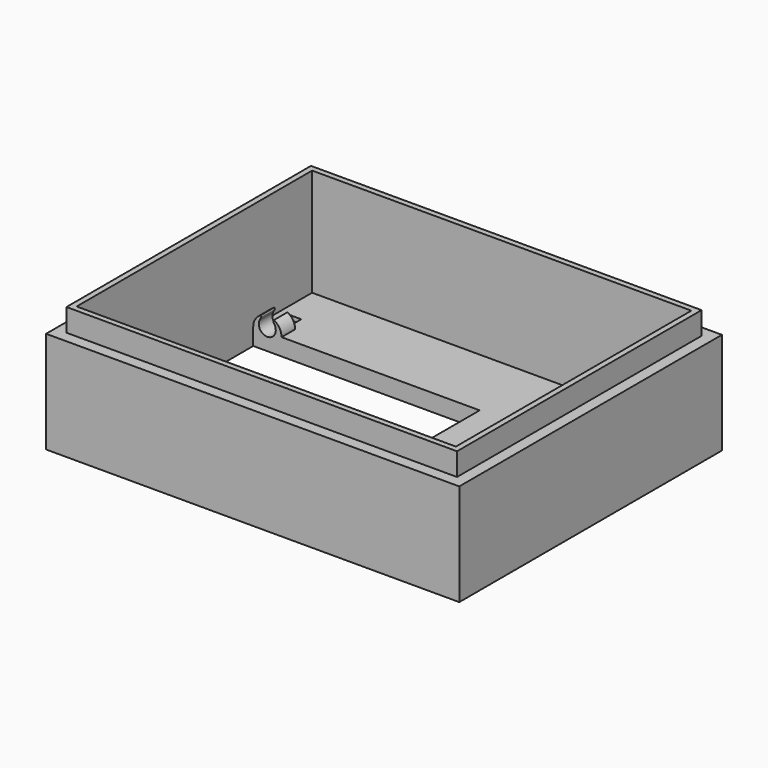
from build123d import *

# Parameters (mm, degrees)
F0_W      = 73
F0_H      = 22
F1_DEPTH  = 29
F2_W      = 67
F2_H      = 52
F3_DEPTH  = 19
F4_W      = 58
F4_H      = 4
F5_DEPTH  = 2
F6_W      = 71
F6_H      = 4
F7_DEPTH  = 2
F8_W      = 56
F8_H      = 4
F9_DEPTH  = 2
F10_W     = 69
F10_H     = 4
F11_DEPTH = 2
F12_W     = 42
F12_H     = 28
F13_DEPTH = 22.001
F14_W     = 2.5
F14_H     = 3
F16_W     = 2.5
F16_H     = 3
F18_R     = 1.5
F19_DEPTH = 35.32766
F20_DEPTH = 5.87666
F22_DEPTH = 38.628
F23_W     = 28
F23_H     = 1.5
F24_DEPTH = 2


with BuildPart() as f1:
    # F0 (on Front) → F1 (new body, symmetric)
    with BuildSketch(Plane.XZ):
        Rectangle(F0_W, F0_H)
    extrude(amount=F1_DEPTH, both=True)

    # F2 (on face) → F3 (cut)
    with BuildSketch(Plane.XY.offset(11)):
        Rectangle(F2_W, F2_H)
    extrude(amount=-F3_DEPTH, mode=Mode.SUBTRACT)

    # F4 (on face) → F5 (cut)
    with BuildSketch(Plane.YZ.offset(36.5)):
        with Locations((0, 9)):
            Rectangle(F4_W, F4_H)
    extrude(amount=-F5_DEPTH, mode=Mode.SUBTRACT)

    # F6 (on face) → F7 (cut)
    with BuildSketch(Plane.XZ.offset(29)):
        with Locations((-1, 9)):
            Rectangle(F6_W, F6_H)
    extrude(amount=-F7_DEPTH, mode=Mode.SUBTRACT)

    # F8 (on face) → F9 (cut)
    with BuildSketch(Plane(origin=(-36.5, 0, 0), x_dir=(0, -1, 0), z_dir=(-1, 0, 0))):
        with Locations((-1, 9)):
            Rectangle(F8_W, F8_H)
    extrude(amount=-F9_DEPTH, mode=Mode.SUBTRACT)

    # F10 (on face) → F11 (cut)
    with BuildSketch(Plane(origin=(0, 29, 0), x_dir=(-1, 0, 0), z_dir=(0, 1, 0))):
        with Locations((0, 9)):
            Rectangle(F10_W, F10_H)
    extrude(amount=-F11_DEPTH, mode=Mode.SUBTRACT)

    # F12 (on face) → F13 (cut, through all)
    with BuildSketch(Plane(origin=(0, 0, -11), x_dir=(1, 0, 0), z_dir=(0, 0, -1))):
        with Locations((-12.5, 1)):
            Rectangle(F12_W, F12_H)
    extrude(amount=-F13_DEPTH, mode=Mode.SUBTRACT)

    # F14 (on face) → F15 (revolve)
    with BuildSketch(Plane.XY.offset(-8)):
        with Locations((-32.25, -16.5)):
            Rectangle(F14_W, F14_H)
    revolve(axis=Axis((-31, -16.5, -8), (0, -1, 0)))

    # F16 (on face) → F17 (revolve)
    with BuildSketch(Plane.XY.offset(-8)):
        with Locations((-32.25, 14.5)):
            Rectangle(F16_W, F16_H)
    revolve(axis=Axis((-31, 14.5, -8), (0, 1, 0)))

    # F18 (on face) → F19 (cut)
    with BuildSketch(Plane.XZ.offset(-13)):
        with Locations((-31.0196849202, -7.260261868)):
            Circle(F18_R)
    extrude(amount=F19_DEPTH, mode=Mode.SUBTRACT)

    # F18 (on face) → F20 (cut)
    with BuildSketch(Plane.XZ.offset(-13)):
        with Locations((-31.0196849202, -7.260261868)):
            Circle(F18_R)
    extrude(amount=-F20_DEPTH, mode=Mode.SUBTRACT)

    # F21 (on face) → F22 (cut)
    with BuildSketch(Plane.XZ.offset(18)):
        with BuildLine():
            add(Edge.make_bspline(
                [(-32.3582060158, -6.5832380305), (-32.2676000125, -6.2528454981), (-31.9089266521, -6.0518947977), (-32.1771532814, -5.7944818858)],
                knots=[0, 0, 0, 0, 0.8092690211, 0.8092690211, 0.8092690211, 0.8092690211], degree=3))
            ThreePointArc((-32.3582060158, -6.5832380305), (-31.0196849202, -5.760261868), (-29.6811638245, -6.5832380305))
            add(Edge.make_bspline(
                [(-29.8511186855, -5.7796235172), (-30.1309504135, -6.0518947977), (-29.7859304255, -6.2528454981), (-29.6811638245, -6.5832380305)],
                knots=[0, 0, 0, 0, 0.82138964, 0.82138964, 0.82138964, 0.82138964], degree=3))
            ThreePointArc((-29.8511186855, -5.7796235172), (-31.0159693083, -5.5000510043), (-32.1771532814, -5.7944818858))
        make_face()
    extrude(amount=-F22_DEPTH, mode=Mode.SUBTRACT)

    # F23 (on face) → F24 (join)
    with BuildSketch(Plane(origin=(8.5, 0, 0), x_dir=(0, -1, 0), z_dir=(-1, 0, 0))):
        with Locations((1, -8.75)):
            Rectangle(F23_W, F23_H)
    extrude(amount=F24_DEPTH)


solid = f1.part
